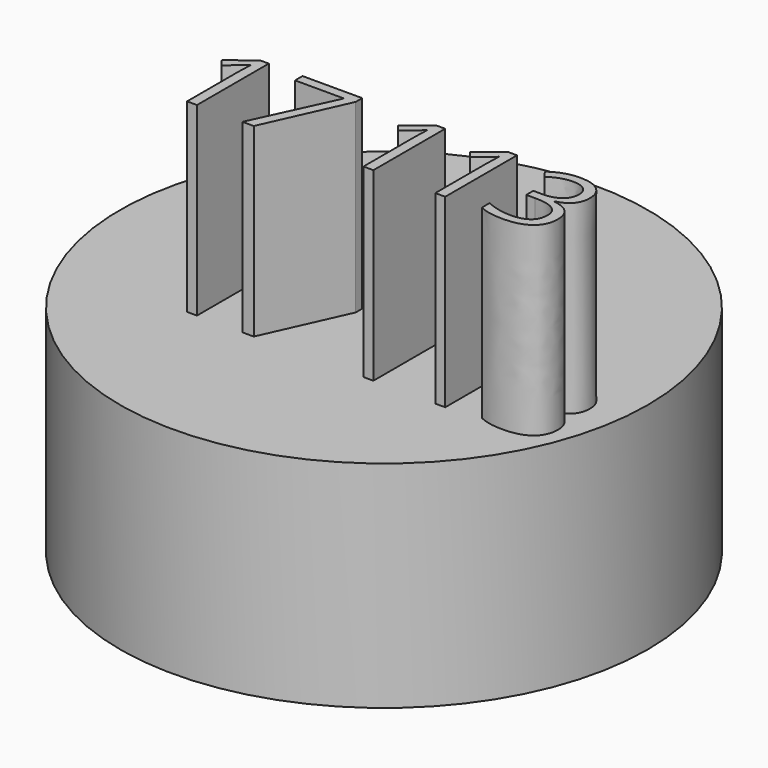
from build123d import *

# Parameters (mm, degrees)
F0_R         = 53.8910215153
F1_DEPTH     = 43.942
F2_TEXT_SIZE = 25.6638561244
F3_DEPTH     = 37.846


# Not quite as in the source:
# - Text() gives the source's letters only with a copy of the font that has no kerning and outlines rounded to 1/6400 em; it was checked with that copy


with BuildPart() as f1:
    # F0 (on Top) → F1 (new body)
    with BuildSketch(Plane.XY):
        with Locations((0, 2.3351607379)):
            Circle(F0_R)
    extrude(amount=F1_DEPTH)

    # F2 (on face) → F3 (join)
    with BuildSketch(Plane.XY.offset(43.942)):
        with Locations((-30.4818178814, -18.4779764096)):
            Text('17 113', F2_TEXT_SIZE, font='Open Sans', text_align=(TextAlign.LEFT, TextAlign.BOTTOM))
    extrude(amount=F3_DEPTH)


solid = f1.part
